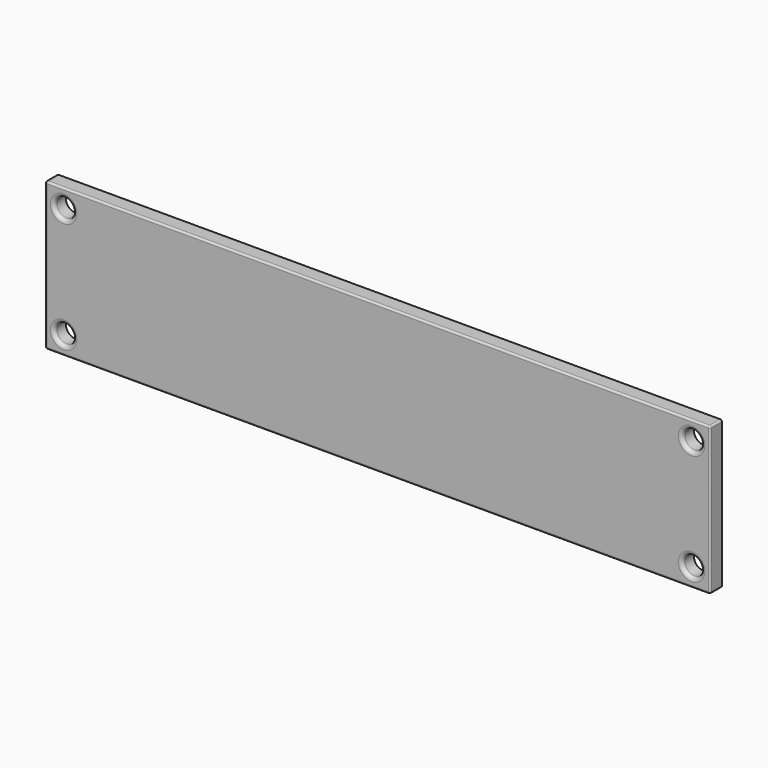
from build123d import *

# Parameters (mm, degrees)
F0_W         = 180
F0_H         = 40
F0_R         = 2.5751263091
F1_DEPTH     = 4
F2_R         = 1
F3_R         = 0.5
F4_TEXT_SIZE = 7.9719321555
F5_DEPTH     = 1


# Not quite as in the source:
# - a feature names something its author has since deleted; it is built from what else it names
# - Text() gives the source's letters only with a copy of the font that has no kerning and outlines rounded to 1/6400 em; it was checked with that copy


with BuildPart() as f1:
    # F0 (on Front) → F1 (new body)
    with BuildSketch(Plane.XZ):
        Rectangle(F0_W, F0_H)
        with Locations((-85, -15)):
            Circle(F0_R, mode=Mode.SUBTRACT)
        with Locations((85, -15)):
            Circle(F0_R, mode=Mode.SUBTRACT)
        with Locations((-85, 15)):
            Circle(F0_R, mode=Mode.SUBTRACT)
        with Locations((85, 15)):
            Circle(F0_R, mode=Mode.SUBTRACT)
    extrude(amount=F1_DEPTH)

    # F2
    f2_edges = [f1.edges().sort_by_distance(p)[0] for p in [
        (-87.575126, -4, 15),
        (-87.575126, -4, -15),
        (82.424874, -4, 15),
        (82.424874, -4, -15),
    ]]
    fillet(f2_edges, radius=F2_R)

    # F3
    f3_edges = [f1.edges().sort_by_distance(p)[0] for p in [
        (0, -4, 20),
        (-90, -4, 0),
        (0, -4, -20),
        (90, -4, 0),
        (-90, -2, 20),
        (-90, -2, -20),
        (90, -2, 20),
        (90, -2, -20),
    ]]
    fillet(f3_edges, radius=F3_R)

    # F4 (on face) → F5 (join)
    with BuildSketch(Plane(origin=(0, 0, 0), x_dir=(-1, 0, 0), z_dir=(0, 1, 0))):
        with Locations((-70.5961091444, -2.9930423558)):
            Text('Havana FP Body', F4_TEXT_SIZE, font='Open Sans', text_align=(TextAlign.LEFT, TextAlign.BOTTOM))
    extrude(amount=F5_DEPTH)

    # F6: F1 across plane


with BuildPart() as f1_1:
    add(f1.part)
    add(f1.part.mirror(Plane.YZ))


solid = f1_1.part
